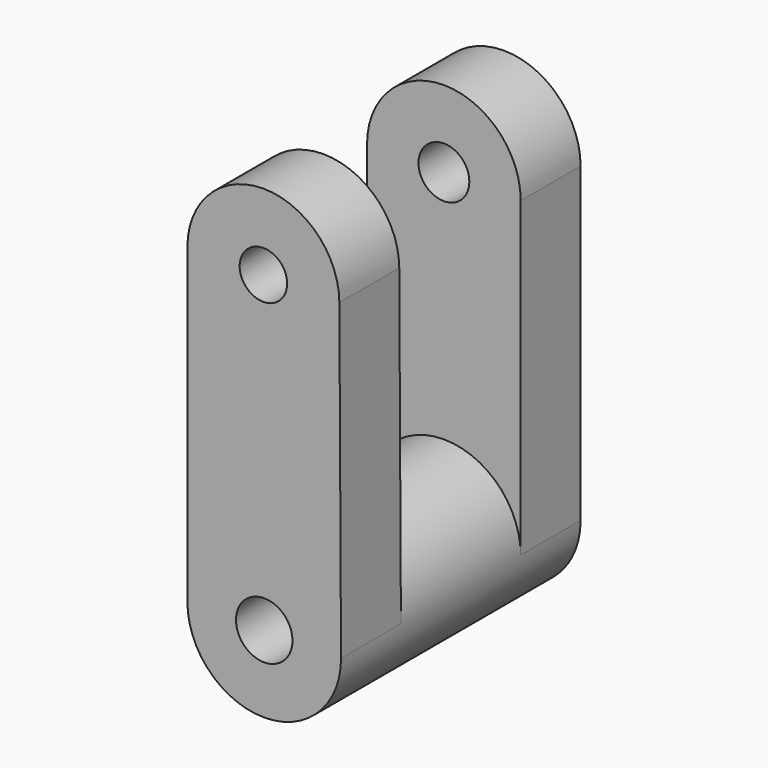
from build123d import *

# Parameters (mm, degrees)
F0_R     = 4.3140137555
F0_R_2   = 4.7914191877
F1_DEPTH = 12.7
F2_DEPTH = 50.8
F3_R     = 4.4074532963
F4_DEPTH = 12.7
F5_R     = 4.030114566
F6_DEPTH = 25.4


# Not quite as in the source:
# - a feature names something its author has since deleted; it is built from what else it names


with BuildPart() as f1:
    # F0 (on Front) → F1 (new body)
    with BuildSketch(Plane.XZ):
        with BuildLine():
            ThreePointArc((9.5125902444, 31.9258160889), (-3.518355079, 44.9567614123), (-16.5493004024, 31.9258160889))
            Line((-16.5493004024, 31.9258160889), (-16.5493004024, -20.979821682))
            ThreePointArc((-16.5493004024, -20.979821682), (-3.518355079, -7.9488763586), (9.5125902444, -20.979821682))
            Line((9.5125902444, -20.979821682), (9.5125902444, 31.9258160889))
        make_face()
        with Locations((-3.518355079, 31.9258160889)):
            Circle(F0_R, mode=Mode.SUBTRACT)
        with BuildLine():
            ThreePointArc((9.5125902444, -20.979821682), (-3.518355079, -7.9488763586), (-16.5493004024, -20.979821682))
            ThreePointArc((-16.5493004024, -20.979821682), (-3.518355079, -34.0107670054), (9.5125902444, -20.979821682))
        make_face()
        with Locations((-3.518355079, -20.979821682)):
            Circle(F0_R_2, mode=Mode.SUBTRACT)
    extrude(amount=F1_DEPTH)

    # F0 (on Front) → F2 (join)
    with BuildSketch(Plane.XZ):
        with BuildLine():
            ThreePointArc((9.5125902444, -20.979821682), (-3.518355079, -7.9488763586), (-16.5493004024, -20.979821682))
            ThreePointArc((-16.5493004024, -20.979821682), (-3.518355079, -34.0107670054), (9.5125902444, -20.979821682))
        make_face()
        with Locations((-3.518355079, -20.979821682)):
            Circle(F0_R_2, mode=Mode.SUBTRACT)
    extrude(amount=F2_DEPTH)

    # F3 (on face) → F4 (join)
    with BuildSketch(Plane.XZ.offset(50.8)):
        with BuildLine():
            Line((-16.5491351407, 32.1166292513), (-16.5491351407, -21.0454494616))
            ThreePointArc((-16.5491351407, -21.0454494616), (-3.5857392287, -7.9490505844), (9.5124068178, -20.9106811633))
            Line((9.5124068178, -20.9106811633), (9.2310467735, 32.1166292513))
            ThreePointArc((9.2310467735, 32.1166292513), (-3.6590441836, 44.9385075287), (-16.5491351407, 32.1166292513))
        make_face()
        with Locations((-3.6590441836, 32.0482351251)):
            Circle(F3_R, mode=Mode.SUBTRACT)
        with Locations((-3.6590441836, 32.0482351251)):
            Circle(F3_R)
    extrude(amount=-F4_DEPTH)

    # F5 (on face) → F6 (cut)
    with BuildSketch(Plane.XZ.offset(50.8)):
        with Locations((-3.6590441836, 32.0482351251)):
            Circle(F5_R)
    extrude(amount=-F6_DEPTH, mode=Mode.SUBTRACT)


solid = f1.part
